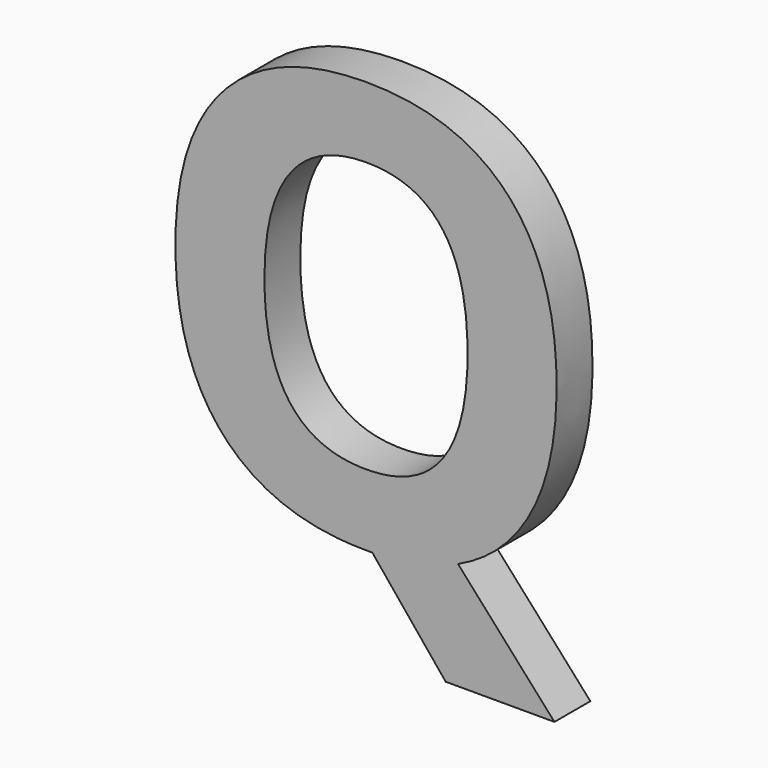
from build123d import *

# Parameters (mm, degrees)
F0_TEXT_SIZE = 62.5
F1_DEPTH     = 5


# Not quite as in the source:
# - Text() gives the source's letters only with a copy of the font that has no kerning and outlines rounded to 1/6400 em; it was checked with that copy


with BuildPart() as f1:
    # F0 (on Front) → F1 (new body)
    with BuildSketch(Plane.XZ):
        with Locations((-55.8149170329, 14.1712714937)):
            Text('Q', F0_TEXT_SIZE, font='Open Sans', font_style=FontStyle.BOLD, text_align=(TextAlign.LEFT, TextAlign.BOTTOM))
    extrude(amount=F1_DEPTH)


solid = f1.part
